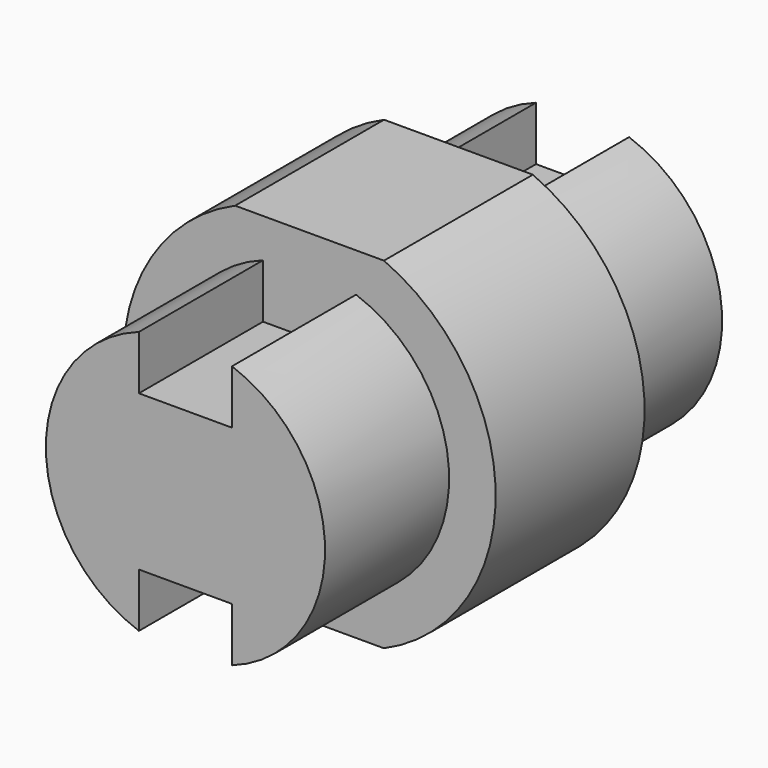
from build123d import *

# Parameters (mm, degrees)
F0_R     = 30
F1_DEPTH = 15
F2_R     = 22.5
F3_DEPTH = 25
F4_R     = 22.5
F5_DEPTH = 25
F6_W     = 30
F6_H     = 8
F7_DEPTH = 15
F8_W     = 15
F8_H     = 12
F9_DEPTH = 25


# Not quite as in the source:
# - a pattern or mirror of a feature is missing from the dataset's text; its kind, count and spacing are read off the source's solid


with BuildPart() as f1:
    # F0 (on Front) → F1 (new body, symmetric)
    with BuildSketch(Plane.XZ):
        Circle(F0_R)
    extrude(amount=F1_DEPTH, both=True)

    # F2 (on face) → F3 (join)
    with BuildSketch(Plane.XZ.offset(15)):
        Circle(F2_R)
    extrude(amount=F3_DEPTH)

    # F4 (on face) → F5 (join)
    with BuildSketch(Plane(origin=(0, 15, 0), x_dir=(-1, 0, 0), z_dir=(0, 1, 0))):
        Circle(F4_R)
    extrude(amount=F5_DEPTH)

    # F6 (on Front) → F7 (cut, symmetric)
    with BuildSketch(Plane.XZ):
        with Locations((0, 31.5)):
            Rectangle(F6_W, F6_H)
        with Locations((0, -31.5)):
            Rectangle(F6_W, F6_H)
    extrude(amount=F7_DEPTH, both=True, mode=Mode.SUBTRACT)

    # F8 (on face) → F9 (cut)
    with BuildSketch(Plane.XZ.offset(40)):
        with Locations((0, 18.5)):
            Rectangle(F8_W, F8_H)
        with Locations((0, -18.5)):
            Rectangle(F8_W, F8_H)
    f9 = extrude(amount=-F9_DEPTH, mode=Mode.SUBTRACT)

    # F9_copies: F9 across plane
    add(f9.mirror(Plane.ZX), mode=Mode.SUBTRACT)


solid = f1.part
